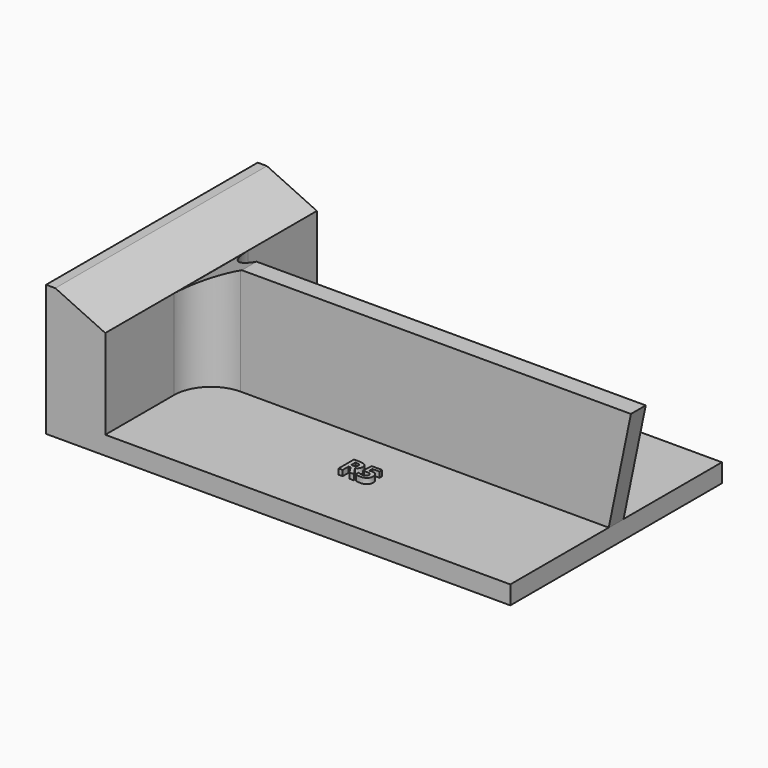
from build123d import *

# Parameters (mm, degrees)
F0_W          = 1.27
F0_H          = 15.494
F1_DEPTH      = 36.322
F4_DEPTH      = 36.322
F5_W          = 55.626
F5_H          = 2.54
F6_DEPTH      = 14.732
F9_DEPTH      = 2.54
F11_DEPTH     = 2.54
F12_TEXT_SIZE = 3.7078823273
F13_DEPTH     = 0.762
F14_R         = 5.08


# Not quite as in the source:
# - Text() gives the source's letters only with a copy of the font that has no kerning and outlines rounded to 1/6400 em; it was checked with that copy


with BuildPart() as f1:
    # F0 (on Front) → F1 (new body)
    with BuildSketch(Plane.XZ):
        Polygon((0, 2.54), (0, 0), (63.754, 0), (63.754, 2.54), (1.27, 2.54), align=None)
        with Locations((0.635, 10.287)):
            Rectangle(F0_W, F0_H)
    extrude(amount=-F1_DEPTH)

    # F3 (on face) → F4 (join)
    with BuildSketch(Plane.XZ):
        Polygon((8.128, 14.8360620804), (1.27, 18.034), (1.27, 2.54), (8.128, 2.54), align=None)
    extrude(amount=-F4_DEPTH)

    # F5 (on face) → F6 (join)
    with BuildSketch(Plane.XY.offset(2.54)):
        with Locations((35.941, 18.161)):
            Rectangle(F5_W, F5_H)
    extrude(amount=F6_DEPTH)

    # F8 (on face) → F9 (cut)
    with BuildSketch(Plane.XZ.offset(-16.891)):
        Polygon((8.128, 17.272), (8.128, 14.8138116455), (13.3739808066, 17.272), align=None)
    extrude(amount=-F9_DEPTH, mode=Mode.SUBTRACT)

    # F10 (on face) → F11 (join)
    with BuildSketch(Plane.XZ.offset(-16.891)):
        Polygon((63.754, 17.272), (63.754, 2.5116572983), (66.802, 17.272), align=None)
    extrude(amount=-F11_DEPTH)

    # F12 (on face) → F13 (join)
    with BuildSketch(Plane.XY.offset(2.54)):
        with Locations((33.1262759864, 8.3792582154)):
            Text('R5', F12_TEXT_SIZE, font='Open Sans', font_style=FontStyle.BOLD, text_align=(TextAlign.LEFT, TextAlign.BOTTOM))
    extrude(amount=F13_DEPTH)

    # F14
    f14_edges = [f1.edges().sort_by_distance(p)[0] for p in [
        (8.128, 16.891, 8.676906),
        (8.128, 19.431, 8.676906),
    ]]
    fillet(f14_edges, radius=F14_R)


solid = f1.part
